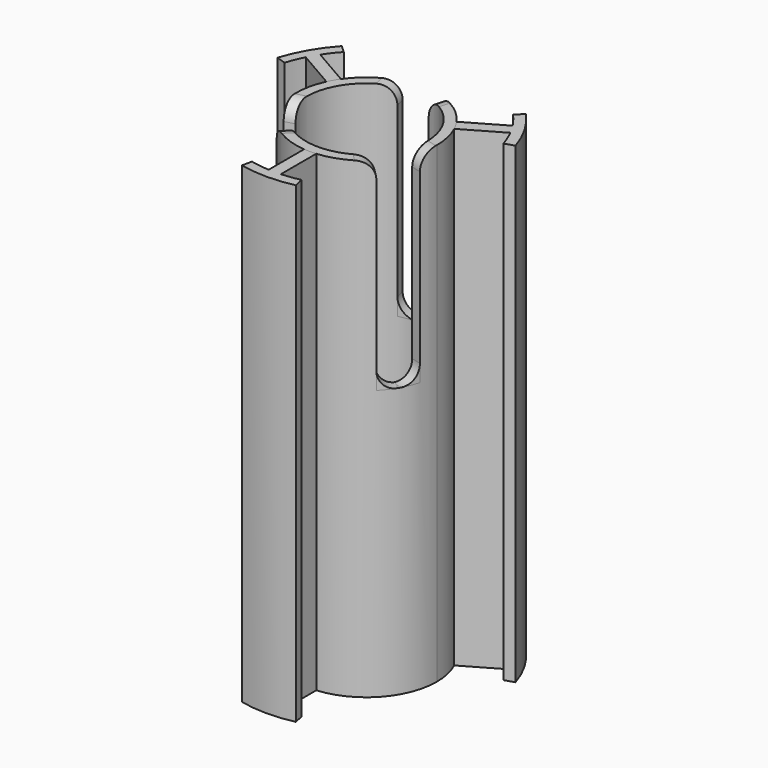
from build123d import *

# Parameters (mm, degrees)
F1_DEPTH     = 70
F0_R         = 8.95
F0_R_2       = 7.45
F2_DEPTH     = 1.2
F3_DEPTH     = 70
F5_DEPTH     = 30
F6_T4_DEPTH  = 14
F6_S5_R      = 10.45
F6_T6_DEPTH  = 10
F6_S7_R      = 8.95
F6_T8_DEPTH  = 10
F6_T12_DEPTH = 14
F6_S13_R     = 10.45
F6_T14_DEPTH = 9
F6_S15_R     = 8.95
F6_T16_DEPTH = 9
F6_T20_DEPTH = 14
F6_S21_R     = 10.45
F6_T22_DEPTH = 9
F6_S23_R     = 8.95
F6_T24_DEPTH = 9
F6_T28_DEPTH = 14
F6_S29_R     = 10.45
F6_T30_DEPTH = 9
F6_S31_R     = 8.95
F6_T32_DEPTH = 9
F6_T36_DEPTH = 14
F6_S37_R     = 10.45
F6_T38_DEPTH = 9
F6_S39_R     = 8.95
F6_T40_DEPTH = 9
F6_T44_DEPTH = 14
F6_S45_R     = 10.45
F6_T46_DEPTH = 10
F6_S47_R     = 8.95
F6_T48_DEPTH = 10
F6_T49_DEPTH = 14
F6_T51_DEPTH = 14
F6_T53_DEPTH = 14
F6_T55_DEPTH = 14
F6_T57_DEPTH = 14
F6_T59_DEPTH = 14


# Not quite as in the source:
# - a fillet or chamfer that OpenCascade refuses, or shapes differently, is made with other operations: its cross-section is extruded or revolved along the edge and cut away or added


with BuildPart() as f1:
    # F0 (on Top) → F1 (new body)
    with BuildSketch(Plane.XY):
        with BuildLine():
            ThreePointArc((-0.9, -16.9761597542), (0, -17), (0.9, -16.9761597542))
            Line((0.9, -16.9761597542), (0.9, -10.4111718841))
            ThreePointArc((0.9, -10.4111718841), (0, -10.45), (-0.9, -10.4111718841))
            Line((-0.9, -10.4111718841), (-0.9, -16.9761597542))
        make_face()
        with BuildLine():
            Line((4.0041328579, -18.0614761317), (3.6794734369, -16.597032121))
            ThreePointArc((3.6794734369, -16.597032121), (2.2975701688, -16.8440247957), (0.9, -16.9761597542))
            ThreePointArc((0.9, -16.9761597542), (0, -17), (-0.9, -16.9761597542))
            ThreePointArc((-0.9, -16.9761597542), (-2.2975701688, -16.8440247957), (-3.6794734369, -16.597032121))
            Line((-3.6794734369, -16.597032121), (-4.0041328579, -18.0614761317))
            ThreePointArc((-4.0041328579, -18.0614761317), (0, -18.5), (4.0041328579, -18.0614761317))
        make_face()
    extrude(amount=F1_DEPTH)


with BuildPart() as f1b:
    # F0 (on Top) → F1, piece 2 (new body)
    with BuildSketch(Plane.XY):
        with BuildLine():
            ThreePointArc((-9.4663393348, 4.4261630786), (-9.0499654695, 5.225), (-8.5663393348, 5.9850088054))
            Line((-8.5663393348, 5.9850088054), (-14.2517856058, 9.2675027405))
            ThreePointArc((-14.2517856058, 9.2675027405), (-14.7224318643, 8.5), (-15.1517856058, 7.7086570137))
            Line((-15.1517856058, 7.7086570137), (-9.4663393348, 4.4261630786))
        make_face()
        with BuildLine():
            Line((-12.5337147258, 11.4850335295), (-13.639630731, 12.4984188409))
            ThreePointArc((-13.639630731, 12.4984188409), (-16.02146997, 9.25), (-17.6437635888, 5.5630572908))
            Line((-17.6437635888, 5.5630572908), (-16.2131881627, 5.1119985916))
            ThreePointArc((-16.2131881627, 5.1119985916), (-15.7361384595, 6.4322582647), (-15.1517856058, 7.7086570137))
            ThreePointArc((-15.1517856058, 7.7086570137), (-14.7224318643, 8.5), (-14.2517856058, 9.2675027405))
            ThreePointArc((-14.2517856058, 9.2675027405), (-13.4385682907, 10.411766531), (-12.5337147258, 11.4850335295))
        make_face()
    extrude(amount=F1_DEPTH)


with BuildPart() as f1c:
    # F0 (on Top) → F1, piece 3 (new body)
    with BuildSketch(Plane.XY):
        with BuildLine():
            Line((9.4663393348, 4.4261630786), (15.1517856058, 7.7086570137))
            ThreePointArc((15.1517856058, 7.7086570137), (14.7224318643, 8.5), (14.2517856058, 9.2675027405))
            Line((14.2517856058, 9.2675027405), (8.5663393348, 5.9850088054))
            ThreePointArc((8.5663393348, 5.9850088054), (9.0499654695, 5.225), (9.4663393348, 4.4261630786))
        make_face()
        with BuildLine():
            ThreePointArc((15.1517856058, 7.7086570137), (15.7361384595, 6.4322582647), (16.2131881627, 5.1119985916))
            Line((16.2131881627, 5.1119985916), (17.6437635888, 5.5630572908))
            ThreePointArc((17.6437635888, 5.5630572908), (16.02146997, 9.25), (13.639630731, 12.4984188409))
            Line((13.639630731, 12.4984188409), (12.5337147258, 11.4850335295))
            ThreePointArc((12.5337147258, 11.4850335295), (13.4385682907, 10.411766531), (14.2517856058, 9.2675027405))
            ThreePointArc((14.2517856058, 9.2675027405), (14.7224318643, 8.5), (15.1517856058, 7.7086570137))
        make_face()
    extrude(amount=F1_DEPTH)


with BuildPart() as f2:
    # F0 (on Top) → F2 (new body)
    with BuildSketch(Plane.XY):
        Circle(F0_R)
        Circle(F0_R_2, mode=Mode.SUBTRACT)
    extrude(amount=F2_DEPTH)


with BuildPart() as f3:
    # F0 (on Top) → F3 (new body)
    with BuildSketch(Plane.XY):
        with BuildLine():
            ThreePointArc((10.45, 0), (10.2011211651, 2.2670745413), (9.4663393348, 4.4261630786))
            ThreePointArc((9.4663393348, 4.4261630786), (9.0499654695, 5.225), (8.5663393348, 5.9850088054))
            ThreePointArc((8.5663393348, 5.9850088054), (0, 10.45), (-8.5663393348, 5.9850088054))
            ThreePointArc((-8.5663393348, 5.9850088054), (-9.0499654695, 5.225), (-9.4663393348, 4.4261630786))
            ThreePointArc((-9.4663393348, 4.4261630786), (-9.0499654695, -5.225), (-0.9, -10.4111718841))
            ThreePointArc((-0.9, -10.4111718841), (0, -10.45), (0.9, -10.4111718841))
            ThreePointArc((0.9, -10.4111718841), (7.7008928054, -7.0639047276), (10.45, 0))
        make_face()
        Circle(F0_R, mode=Mode.SUBTRACT)
    extrude(amount=F3_DEPTH)

    # F4 (on face) → F5 (cut)
    with BuildSketch(Plane.XY.offset(70)):
        with BuildLine():
            Line((-7.3892658634, -7.3892658634), (-6.3286056916, -6.3286056916))
            ThreePointArc((-6.3286056916, -6.3286056916), (-7.7509273639, -4.475), (-8.6450361453, -2.3164304537))
            Line((-8.6450361453, -2.3164304537), (-10.0939248847, -2.7046590213))
            ThreePointArc((-10.0939248847, -2.7046590213), (-9.0499654695, -5.225), (-7.3892658634, -7.3892658634))
        make_face()
        with BuildLine():
            Line((10.0939248847, -2.7046590213), (8.6450361453, -2.3164304537))
            ThreePointArc((8.6450361453, -2.3164304537), (7.7509273639, -4.475), (6.3286056916, -6.3286056916))
            Line((6.3286056916, -6.3286056916), (7.3892658634, -7.3892658634))
            ThreePointArc((7.3892658634, -7.3892658634), (9.0499654695, -5.225), (10.0939248847, -2.7046590213))
        make_face()
        with BuildLine():
            ThreePointArc((-2.3164304537, 8.6450361453), (0, 8.95), (2.3164304537, 8.6450361453))
            Line((2.3164304537, 8.6450361453), (2.7046590213, 10.0939248847))
            ThreePointArc((2.7046590213, 10.0939248847), (0, 10.45), (-2.7046590213, 10.0939248847))
            Line((-2.7046590213, 10.0939248847), (-2.3164304537, 8.6450361453))
        make_face()
    extrude(amount=-F5_DEPTH, mode=Mode.SUBTRACT)

    # F6: fillet of radius 2.5 on 12 edges, made by hand


with BuildPart() as f6_tool2:
    # F6_s3 → F6_t4 (new body)
    with BuildSketch(Plane(origin=(-11.8086832458, -11.8086832458, 0), x_dir=(0, 0, 1), z_dir=(0.7071067812, 0.7071067812, 0))):
        with BuildLine():
            ThreePointArc((42.5, 0), (40.732233047, -0.732233047), (40, -2.5))
            Line((40, -2.5), (40, 0))
            Line((40, 0), (42.5, 0))
        make_face()
    extrude(amount=F6_T4_DEPTH)

    # F6_s5 → F6_t6 (intersect, symmetric)
    with BuildSketch(Plane.XY.offset(41.2)):
        Circle(F6_S5_R)
    extrude(amount=F6_T6_DEPTH, both=True, mode=Mode.INTERSECT)

    # F6_s7 → F6_t8 (cut, symmetric)
    with BuildSketch(Plane.XY.offset(41.2)):
        Circle(F6_S7_R)
    extrude(amount=F6_T8_DEPTH, both=True, mode=Mode.SUBTRACT)


with BuildPart() as f3_1:
    add(f3.part)

    # F6_t1: union F6_tool2
    add(f6_tool2.part)


with BuildPart() as f6_tool10:
    # F6_s11 → F6_t12 (new body)
    with BuildSketch(Plane(origin=(-2.607999731, -0.6988114218, 0), x_dir=(0, 0, 1), z_dir=(-0.9659258263, -0.2588190451, 0))):
        with BuildLine():
            ThreePointArc((40, -2.5), (40.732233047, -0.732233047), (42.5, 0))
            Line((42.5, 0), (40, 0))
            Line((40, 0), (40, -2.5))
        make_face()
    extrude(amount=F6_T12_DEPTH)

    # F6_s13 → F6_t14 (intersect, symmetric)
    with BuildSketch(Plane.XY.offset(41.2)):
        Circle(F6_S13_R)
    extrude(amount=F6_T14_DEPTH, both=True, mode=Mode.INTERSECT)

    # F6_s15 → F6_t16 (cut, symmetric)
    with BuildSketch(Plane.XY.offset(41.2)):
        Circle(F6_S15_R)
    extrude(amount=F6_T16_DEPTH, both=True, mode=Mode.SUBTRACT)


with BuildPart() as f3_2:
    add(f3_1.part)

    # F6_t9: union F6_tool10
    add(f6_tool10.part)


with BuildPart() as f6_tool18:
    # F6_s19 → F6_t20 (new body)
    with BuildSketch(Plane(origin=(-4.3222780532, 16.130961299, 0), x_dir=(0, 0, 1), z_dir=(0.2588190451, -0.9659258263, 0))):
        with BuildLine():
            ThreePointArc((42.5, 0), (40.732233047, -0.732233047), (40, -2.5))
            Line((40, -2.5), (40, 0))
            Line((40, 0), (42.5, 0))
        make_face()
    extrude(amount=F6_T20_DEPTH)

    # F6_s21 → F6_t22 (intersect, symmetric)
    with BuildSketch(Plane.XY.offset(41.2)):
        Circle(F6_S21_R)
    extrude(amount=F6_T22_DEPTH, both=True, mode=Mode.INTERSECT)

    # F6_s23 → F6_t24 (cut, symmetric)
    with BuildSketch(Plane.XY.offset(41.2)):
        Circle(F6_S23_R)
    extrude(amount=F6_T24_DEPTH, both=True, mode=Mode.SUBTRACT)


with BuildPart() as f3_3:
    add(f3_2.part)

    # F6_t17: union F6_tool18
    add(f6_tool18.part)


with BuildPart() as f6_tool26:
    # F6_s27 → F6_t28 (new body)
    with BuildSketch(Plane(origin=(0.6988114218, 2.607999731, 0), x_dir=(0, 0, 1), z_dir=(0.2588190451, 0.9659258263, 0))):
        with BuildLine():
            ThreePointArc((40, -2.5), (40.732233047, -0.732233047), (42.5, 0))
            Line((42.5, 0), (40, 0))
            Line((40, 0), (40, -2.5))
        make_face()
    extrude(amount=F6_T28_DEPTH)

    # F6_s29 → F6_t30 (intersect, symmetric)
    with BuildSketch(Plane.XY.offset(41.2)):
        Circle(F6_S29_R)
    extrude(amount=F6_T30_DEPTH, both=True, mode=Mode.INTERSECT)

    # F6_s31 → F6_t32 (cut, symmetric)
    with BuildSketch(Plane.XY.offset(41.2)):
        Circle(F6_S31_R)
    extrude(amount=F6_T32_DEPTH, both=True, mode=Mode.SUBTRACT)


with BuildPart() as f3_4:
    add(f3_3.part)

    # F6_t25: union F6_tool26
    add(f6_tool26.part)


with BuildPart() as f6_tool34:
    # F6_s35 → F6_t36 (new body)
    with BuildSketch(Plane(origin=(16.130961299, -4.3222780532, 0), x_dir=(0, 0, 1), z_dir=(-0.9659258263, 0.2588190451, 0))):
        with BuildLine():
            ThreePointArc((42.5, 0), (40.732233047, -0.732233047), (40, -2.5))
            Line((40, -2.5), (40, 0))
            Line((40, 0), (42.5, 0))
        make_face()
    extrude(amount=F6_T36_DEPTH)

    # F6_s37 → F6_t38 (intersect, symmetric)
    with BuildSketch(Plane.XY.offset(41.2)):
        Circle(F6_S37_R)
    extrude(amount=F6_T38_DEPTH, both=True, mode=Mode.INTERSECT)

    # F6_s39 → F6_t40 (cut, symmetric)
    with BuildSketch(Plane.XY.offset(41.2)):
        Circle(F6_S39_R)
    extrude(amount=F6_T40_DEPTH, both=True, mode=Mode.SUBTRACT)


with BuildPart() as f3_5:
    add(f3_4.part)

    # F6_t33: union F6_tool34
    add(f6_tool34.part)


with BuildPart() as f6_tool42:
    # F6_s43 → F6_t44 (new body)
    with BuildSketch(Plane(origin=(1.9091883092, -1.9091883092, 0), x_dir=(0, 0, 1), z_dir=(0.7071067812, -0.7071067812, 0))):
        with BuildLine():
            ThreePointArc((40, -2.5), (40.732233047, -0.732233047), (42.5, 0))
            Line((42.5, 0), (40, 0))
            Line((40, 0), (40, -2.5))
        make_face()
    extrude(amount=F6_T44_DEPTH)

    # F6_s45 → F6_t46 (intersect, symmetric)
    with BuildSketch(Plane.XY.offset(41.2)):
        Circle(F6_S45_R)
    extrude(amount=F6_T46_DEPTH, both=True, mode=Mode.INTERSECT)

    # F6_s47 → F6_t48 (cut, symmetric)
    with BuildSketch(Plane.XY.offset(41.2)):
        Circle(F6_S47_R)
    extrude(amount=F6_T48_DEPTH, both=True, mode=Mode.SUBTRACT)


with BuildPart() as f3_6:
    add(f3_5.part)

    # F6_t41: union F6_tool42
    add(f6_tool42.part)

    # F6_s50 → F6_t49 (cut)
    with BuildSketch(Plane(origin=(-11.8086832458, -11.8086832458, 0), x_dir=(0, 0, 1), z_dir=(0.7071067812, 0.7071067812, 0))):
        with BuildLine():
            ThreePointArc((70, 2.5), (69.267766953, 0.732233047), (67.5, 0))
            Line((67.5, 0), (70, 0))
            Line((70, 0), (70, 2.5))
        make_face()
    extrude(amount=F6_T49_DEPTH, mode=Mode.SUBTRACT)

    # F6_s52 → F6_t51 (cut)
    with BuildSketch(Plane(origin=(1.9091883092, -1.9091883092, 0), x_dir=(0, 0, 1), z_dir=(0.7071067812, -0.7071067812, 0))):
        with BuildLine():
            ThreePointArc((70, 2.5), (69.267766953, 0.732233047), (67.5, 0))
            Line((67.5, 0), (70, 0))
            Line((70, 0), (70, 2.5))
        make_face()
    extrude(amount=F6_T51_DEPTH, mode=Mode.SUBTRACT)

    # F6_s54 → F6_t53 (cut)
    with BuildSketch(Plane(origin=(-2.607999731, -0.6988114218, 0), x_dir=(0, 0, 1), z_dir=(-0.9659258263, -0.2588190451, 0))):
        with BuildLine():
            ThreePointArc((67.5, 0), (69.267766953, 0.732233047), (70, 2.5))
            Line((70, 2.5), (70, 0))
            Line((70, 0), (67.5, 0))
        make_face()
    extrude(amount=F6_T53_DEPTH, mode=Mode.SUBTRACT)

    # F6_s56 → F6_t55 (cut)
    with BuildSketch(Plane(origin=(-4.3222780532, 16.130961299, 0), x_dir=(0, 0, 1), z_dir=(0.2588190451, -0.9659258263, 0))):
        with BuildLine():
            ThreePointArc((70, 2.5), (69.267766953, 0.732233047), (67.5, 0))
            Line((67.5, 0), (70, 0))
            Line((70, 0), (70, 2.5))
        make_face()
    extrude(amount=F6_T55_DEPTH, mode=Mode.SUBTRACT)

    # F6_s58 → F6_t57 (cut)
    with BuildSketch(Plane(origin=(0.6988114218, 2.607999731, 0), x_dir=(0, 0, 1), z_dir=(0.2588190451, 0.9659258263, 0))):
        with BuildLine():
            ThreePointArc((67.5, 0), (69.267766953, 0.732233047), (70, 2.5))
            Line((70, 2.5), (70, 0))
            Line((70, 0), (67.5, 0))
        make_face()
    extrude(amount=F6_T57_DEPTH, mode=Mode.SUBTRACT)

    # F6_s60 → F6_t59 (cut)
    with BuildSketch(Plane(origin=(16.130961299, -4.3222780532, 0), x_dir=(0, 0, 1), z_dir=(-0.9659258263, 0.2588190451, 0))):
        with BuildLine():
            ThreePointArc((70, 2.5), (69.267766953, 0.732233047), (67.5, 0))
            Line((67.5, 0), (70, 0))
            Line((70, 0), (70, 2.5))
        make_face()
    extrude(amount=F6_T59_DEPTH, mode=Mode.SUBTRACT)


solid = Compound([f1.part, f1b.part, f1c.part, f2.part, f3_6.part])
